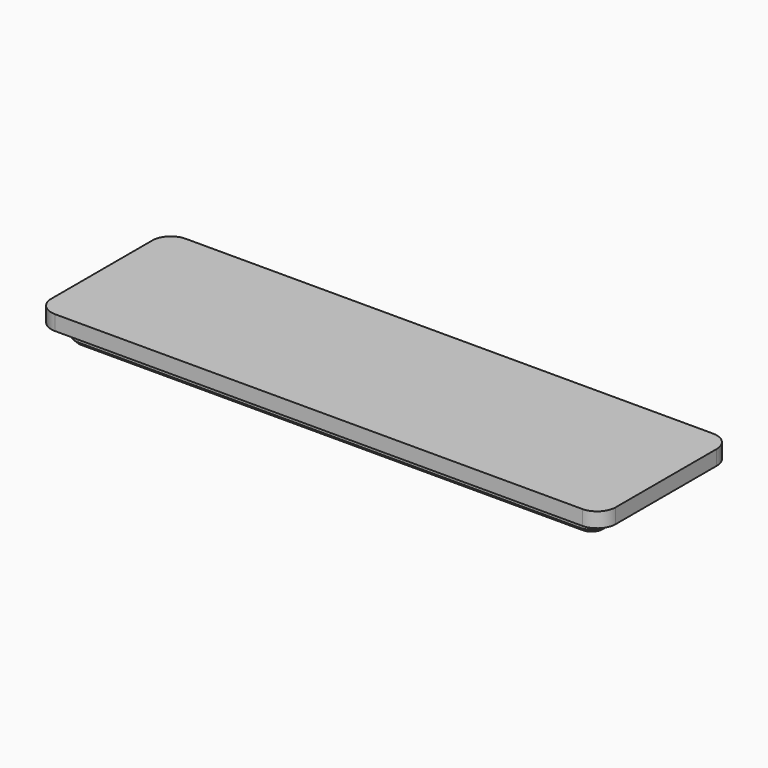
from build123d import *

# Parameters (mm, degrees)
F1_DEPTH     = 2
F2_DEPTH     = 2
F3_SIZE      = 0.5
F4_TEXT_SIZE = 17.7540842237
F5_DEPTH     = 1


# Not quite as in the source:
# - Text() gives the source's letters only with a copy of the font that has no kerning and outlines rounded to 1/6400 em; it was checked with that copy


with BuildPart() as f1:
    # F0 (on Top) → F1 (new body)
    with BuildSketch(Plane.XY):
        with BuildLine():
            Line((-35.5, -11), (35.5, -11))
            ThreePointArc((35.5, -11), (37.267766953, -10.267766953), (38, -8.5))
            Line((38, -8.5), (38, 8.5))
            ThreePointArc((38, 8.5), (37.267766953, 10.267766953), (35.5, 11))
            Line((35.5, 11), (-35.5, 11))
            ThreePointArc((-35.5, 11), (-37.267766953, 10.267766953), (-38, 8.5))
            Line((-38, 8.5), (-38, -8.5))
            ThreePointArc((-38, -8.5), (-37.267766953, -10.267766953), (-35.5, -11))
        make_face()
        with BuildLine():
            ThreePointArc((35.75, -7.25), (35.1642135624, -8.6642135624), (33.75, -9.25))
            Line((33.75, -9.25), (-33.75, -9.25))
            ThreePointArc((-33.75, -9.25), (-35.1642135624, -8.6642135624), (-35.75, -7.25))
            Line((-35.75, -7.25), (-35.75, 7.25))
            ThreePointArc((-35.75, 7.25), (-35.1642135624, 8.6642135624), (-33.75, 9.25))
            Line((-33.75, 9.25), (33.75, 9.25))
            ThreePointArc((33.75, 9.25), (35.1642135624, 8.6642135624), (35.75, 7.25))
            Line((35.75, 7.25), (35.75, -7.25))
        make_face(mode=Mode.SUBTRACT)
        with BuildLine():
            Line((-33.75, -9.25), (33.75, -9.25))
            ThreePointArc((33.75, -9.25), (35.1642135624, -8.6642135624), (35.75, -7.25))
            Line((35.75, -7.25), (35.75, 7.25))
            ThreePointArc((35.75, 7.25), (35.1642135624, 8.6642135624), (33.75, 9.25))
            Line((33.75, 9.25), (-33.75, 9.25))
            ThreePointArc((-33.75, 9.25), (-35.1642135624, 8.6642135624), (-35.75, 7.25))
            Line((-35.75, 7.25), (-35.75, -7.25))
            ThreePointArc((-35.75, -7.25), (-35.1642135624, -8.6642135624), (-33.75, -9.25))
        make_face()
        with BuildLine():
            ThreePointArc((33.75, 7.75), (34.1035533906, 7.6035533906), (34.25, 7.25))
            Line((34.25, 7.25), (34.25, -7.25))
            ThreePointArc((34.25, -7.25), (34.1035533906, -7.6035533906), (33.75, -7.75))
            Line((33.75, -7.75), (-33.75, -7.75))
            ThreePointArc((-33.75, -7.75), (-34.1035533906, -7.6035533906), (-34.25, -7.25))
            Line((-34.25, -7.25), (-34.25, 7.25))
            ThreePointArc((-34.25, 7.25), (-34.1035533906, 7.6035533906), (-33.75, 7.75))
            Line((-33.75, 7.75), (33.75, 7.75))
        make_face(mode=Mode.SUBTRACT)
        with BuildLine():
            Line((34.25, -7.25), (34.25, 7.25))
            ThreePointArc((34.25, 7.25), (34.1035533906, 7.6035533906), (33.75, 7.75))
            Line((33.75, 7.75), (-33.75, 7.75))
            ThreePointArc((-33.75, 7.75), (-34.1035533906, 7.6035533906), (-34.25, 7.25))
            Line((-34.25, 7.25), (-34.25, -7.25))
            ThreePointArc((-34.25, -7.25), (-34.1035533906, -7.6035533906), (-33.75, -7.75))
            Line((-33.75, -7.75), (33.75, -7.75))
            ThreePointArc((33.75, -7.75), (34.1035533906, -7.6035533906), (34.25, -7.25))
        make_face()
    extrude(amount=F1_DEPTH)

    # F0 (on Top) → F2 (join)
    with BuildSketch(Plane.XY):
        with BuildLine():
            Line((-33.75, -9.25), (33.75, -9.25))
            ThreePointArc((33.75, -9.25), (35.1642135624, -8.6642135624), (35.75, -7.25))
            Line((35.75, -7.25), (35.75, 7.25))
            ThreePointArc((35.75, 7.25), (35.1642135624, 8.6642135624), (33.75, 9.25))
            Line((33.75, 9.25), (-33.75, 9.25))
            ThreePointArc((-33.75, 9.25), (-35.1642135624, 8.6642135624), (-35.75, 7.25))
            Line((-35.75, 7.25), (-35.75, -7.25))
            ThreePointArc((-35.75, -7.25), (-35.1642135624, -8.6642135624), (-33.75, -9.25))
        make_face()
        with BuildLine():
            ThreePointArc((33.75, 7.75), (34.1035533906, 7.6035533906), (34.25, 7.25))
            Line((34.25, 7.25), (34.25, -7.25))
            ThreePointArc((34.25, -7.25), (34.1035533906, -7.6035533906), (33.75, -7.75))
            Line((33.75, -7.75), (-33.75, -7.75))
            ThreePointArc((-33.75, -7.75), (-34.1035533906, -7.6035533906), (-34.25, -7.25))
            Line((-34.25, -7.25), (-34.25, 7.25))
            ThreePointArc((-34.25, 7.25), (-34.1035533906, 7.6035533906), (-33.75, 7.75))
            Line((-33.75, 7.75), (33.75, 7.75))
        make_face(mode=Mode.SUBTRACT)
    extrude(amount=-F2_DEPTH)

    # F3
    f3_edges = [f1.edges().sort_by_distance(p)[0] for p in [
        (0, 9.25, -2),
    ]]
    chamfer(f3_edges, length=F3_SIZE)

    # F4 (on face) → F5 (cut)
    with BuildSketch(Plane(origin=(0, 0, 0), x_dir=(1, 0, 0), z_dir=(0, 0, -1))):
        with Locations((-16.0424795415, -6.4445286989)):
            Text('Ben', F4_TEXT_SIZE, font='Open Sans', text_align=(TextAlign.LEFT, TextAlign.BOTTOM))
    extrude(amount=-F5_DEPTH, mode=Mode.SUBTRACT)


solid = f1.part
